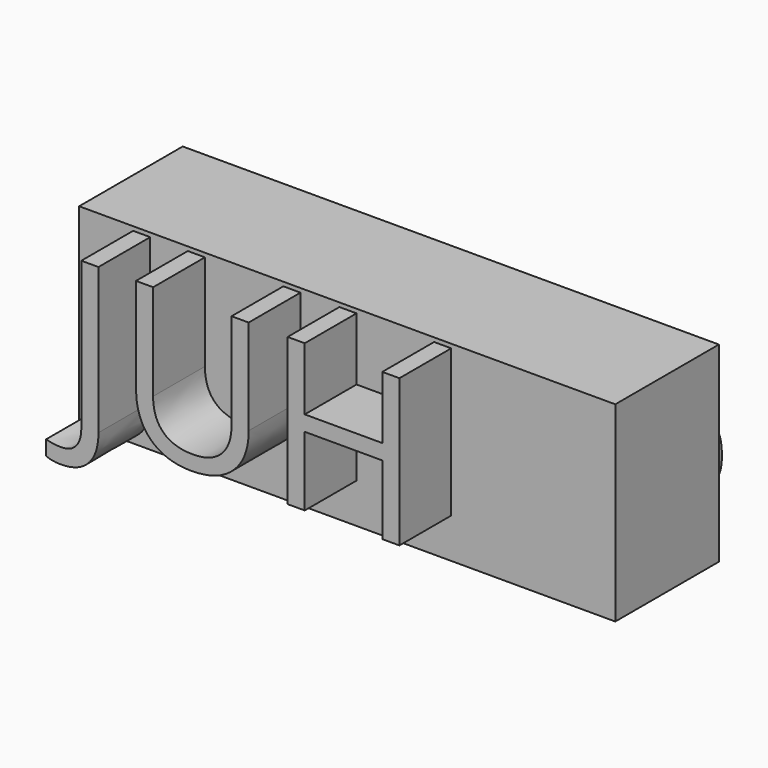
from build123d import *

# Parameters (mm, degrees)
F0_W         = 105.1744371653
F0_H         = 37.5162102282
F1_DEPTH     = 25.4
F2_TEXT_SIZE = 40.4556453254
F3_DEPTH     = 12.7
F5_TEXT_SIZE = 14.9785444476
F6_DEPTH     = 12.7
F7_DEPTH     = 12.7


# Not quite as in the source:
# - Text() gives the source's letters only with a copy of the font that has no kerning and outlines rounded to 1/6400 em; it was checked with that copy


with BuildPart() as f1:
    # F0 (on Front) → F1 (new body)
    with BuildSketch(Plane.XZ):
        with Locations((52.5872185826, 18.7581051141)):
            Rectangle(F0_W, F0_H)
    extrude(amount=F1_DEPTH)

    # F2 (on face) → F3 (join)
    with BuildSketch(Plane.XZ.offset(25.4)):
        with Locations((6.8350352813, 7.8350823605)):
            Text('JUH', F2_TEXT_SIZE, font='Open Sans', text_align=(TextAlign.LEFT, TextAlign.BOTTOM))
    extrude(amount=F3_DEPTH)

    # F5 (on face) → F6 (join)
    with BuildSketch(Plane(origin=(0, 0, 0), x_dir=(-1, 0, 0), z_dir=(0, 1, 0))):
        with Locations((-96.3618879905, 4.7186808661)):
            Text('01055119673', F5_TEXT_SIZE, font='Open Sans', text_align=(TextAlign.LEFT, TextAlign.BOTTOM))
    extrude(amount=F6_DEPTH)

    # F5 (on face) → F7 (join)
    with BuildSketch(Plane(origin=(0, 0, 0), x_dir=(-1, 0, 0), z_dir=(0, 1, 0))):
        with Locations((-96.3618879905, 4.7186808661)):
            Text('01055119673', F5_TEXT_SIZE, font='Open Sans', text_align=(TextAlign.LEFT, TextAlign.BOTTOM))
    extrude(amount=F7_DEPTH)


solid = f1.part
